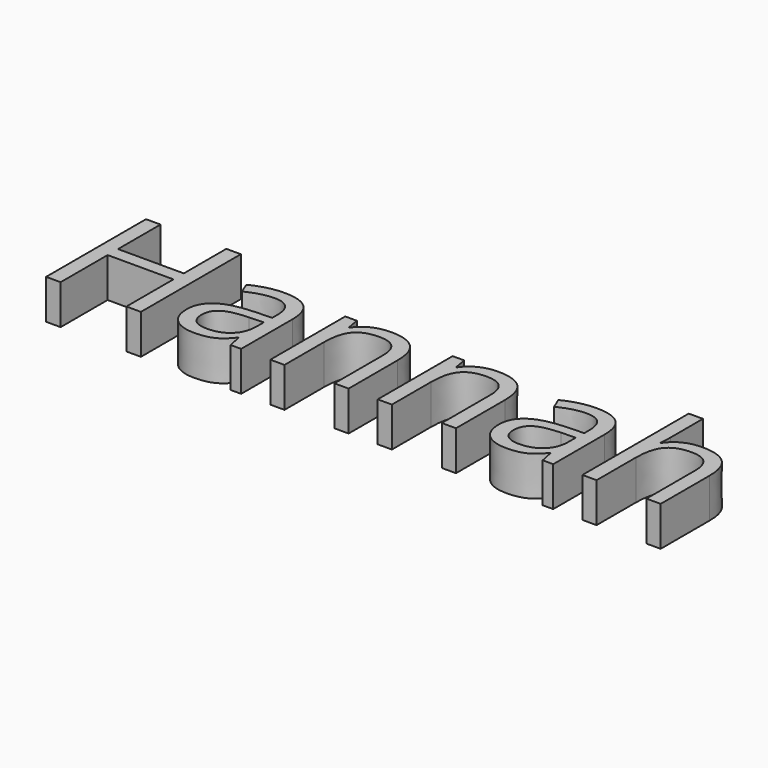
from build123d import *

# Parameters (mm, degrees)
F0_TEXT_SIZE = 36.2387056359
F1_DEPTH     = 8.2


# Not quite as in the source:
# - Text() gives the source's letters only with a copy of the font that has no kerning and outlines rounded to 1/6400 em; it was checked with that copy


with BuildPart() as f1:
    # F0 (on Top) → F1 (new body)
    with BuildSketch(Plane.XY):
        with Locations((-67.7202641964, 8.1833582371)):
            Text('Hannah', F0_TEXT_SIZE, font='Open Sans', text_align=(TextAlign.LEFT, TextAlign.BOTTOM))
    extrude(amount=F1_DEPTH)


solid = f1.part
